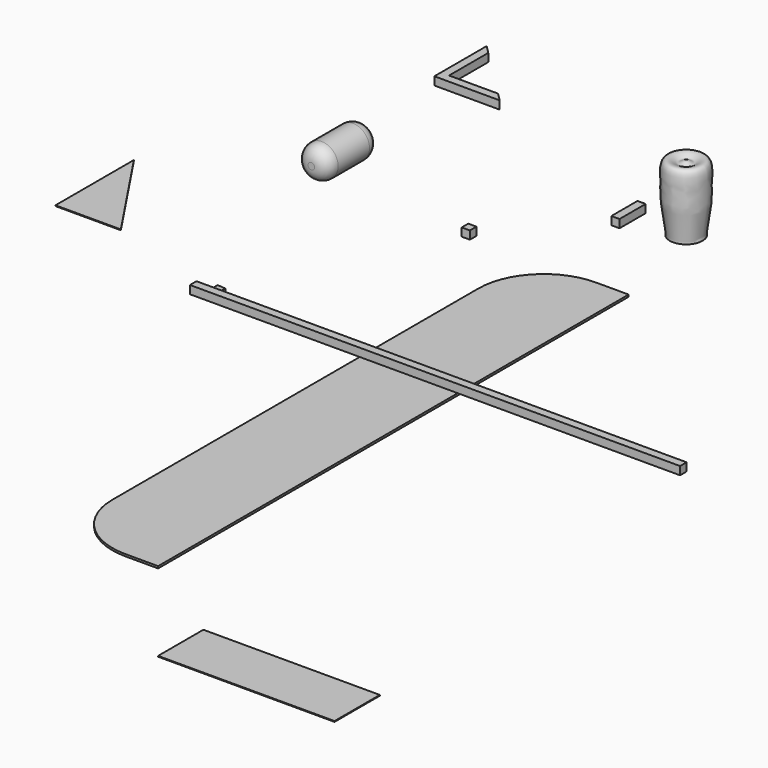
from build123d import *

# Parameters (mm, degrees)
F0_W      = 76.2
F0_H      = 1.5875
F1_DEPTH  = 457.2
F2_W      = 6.35
F2_H      = 6.35
F3_DEPTH  = 381
F4_W      = 44.45
F4_H      = 6.35
F5_DEPTH  = 6.35
F6_SIZE2  = 6.34999
F6_SIZE   = 6.34999
F7_SIZE2  = 6.34999
F7_SIZE   = 6.34999
F8_ANGLE  = 90
F9_W      = 6.35
F9_H      = 6.35
F10_DEPTH = 6.35
F11_R     = 50.8
F12_R     = 50.8
F13_W     = 137.16
F13_H     = 44.0000009
F14_DEPTH = 0.5999999938
F15_W     = 6.35
F15_H     = 6.35
F16_DEPTH = 25.4
F18_DEPTH = 0.5999999938
F20_DEPTH = 6.35
F21_R     = 12.7
F22_DEPTH = 50.8
F23_R     = 10.16
F24_R     = 10.16


# Not quite as in the source:
# - a fillet or chamfer is up to 0.001 mm smaller than in the source, because OpenCascade refuses the exact size


with BuildPart() as f1:
    # F0 (on Front) → F1 (new body)
    with BuildSketch(Plane.XZ):
        with Locations((27.2368646166, 23.0428799987)):
            Rectangle(F0_W, F0_H)
    extrude(amount=F1_DEPTH)

    # F11
    f11_edges = [f1.edges().sort_by_distance(p)[0] for p in [
        (-10.863135, -457.2, 23.04288),
    ]]
    fillet(f11_edges, radius=F11_R)

    # F12
    f12_edges = [f1.edges().sort_by_distance(p)[0] for p in [
        (-10.863135, 0, 23.04288),
    ]]
    fillet(f12_edges, radius=F12_R)


with BuildPart() as f3:
    # F2 (on Right) → F3 (new body)
    with BuildSketch(Plane.YZ):
        with Locations((-341.438638593, 146.0574641824)):
            Rectangle(F2_W, F2_H)
    extrude(amount=F3_DEPTH)


with BuildPart() as f5:
    # F4 (on Front) → F5 (new body)
    with BuildSketch(Plane.XZ):
        with Locations((-52.0163912032, 118.8257239481)):
            Rectangle(F4_W, F4_H)
        Polygon((-74.2413912032, 122.0007239481), (-80.5913912032, 122.0007239481), (-80.5913912032, 71.2007239481), (-74.2413912032, 71.2007239481), (-74.2413912032, 115.6507239481), align=None)
    extrude(amount=F5_DEPTH)

    # F6 (size 6.35 and 6.35 in the source; OpenCascade refuses exactly that, so slightly less here)
    f6_edges = [f5.edges().sort_by_distance(p)[0] for p in [
        (-29.791391, -3.175, 115.650724),
    ]]
    chamfer(f6_edges, length=F6_SIZE, length2=F6_SIZE2)

    # F7 (size 6.35 and 6.35 in the source; OpenCascade refuses exactly that, so slightly less here)
    f7_edges = [f5.edges().sort_by_distance(p)[0] for p in [
        (-74.241391, -3.175, 71.200724),
    ]]
    chamfer(f7_edges, length=F7_SIZE, length2=F7_SIZE2)


with BuildPart() as f5_1:
    # F8: moved
    add(f5.part.rotate(Axis((-55.1913912032, -6.35, 122.0007239481), (1, 0, 0)), F8_ANGLE))


with BuildPart() as f10:
    # F9 (on Front) → F10 (new body)
    with BuildSketch(Plane.XZ):
        with Locations((-56.1577156186, 28.6541397465)):
            Rectangle(F9_W, F9_H)
    extrude(amount=F10_DEPTH)


with BuildPart() as f14:
    # F13 (on Top) → F14 (new body)
    with BuildSketch(Plane.XY):
        with Locations((179.7031573951, -492.4447879232)):
            Rectangle(F13_W, F13_H)
    extrude(amount=F14_DEPTH)


with BuildPart() as f16:
    # F15 (on Front) → F16 (new body)
    with BuildSketch(Plane.XZ):
        with Locations((75.4093378782, 86.979034377)):
            Rectangle(F15_W, F15_H)
    extrude(amount=F16_DEPTH)


with BuildPart() as f18:
    # F17 (on Top) → F18 (new body)
    with BuildSketch(Plane.XY):
        Polygon((-307.5355387568, -14.609475274), (-307.5355387568, -90.809475274), (-256.7355387568, -90.809475274), align=None)
    extrude(amount=F18_DEPTH)


with BuildPart() as f20:
    # F19 (on Top) → F20 (new body)
    with BuildSketch(Plane.XY):
        Polygon((-158.2077033869, -119.8694149069), (-158.2077033869, -126.2194149069), (-151.8577033869, -126.2194149069), (-151.8577033869, -120.4249679203), align=None)
    extrude(amount=F20_DEPTH)


with BuildPart() as f22:
    # F21 (on Front) → F22 (new body)
    with BuildSketch(Plane.XZ):
        with Locations((-140.6690627337, 65.3587505221)):
            Circle(F21_R)
    extrude(amount=F22_DEPTH)

    # F23
    f23_edges = [f22.edges().sort_by_distance(p)[0] for p in [
        (-153.369063, -50.8, 65.358751),
    ]]
    fillet(f23_edges, radius=F23_R)

    # F24
    f24_edges = [f22.edges().sort_by_distance(p)[0] for p in [
        (-153.369063, 0, 65.358751),
    ]]
    fillet(f24_edges, radius=F24_R)


with BuildPart() as f26:
    # F25 (on Front) → F26 (revolve)
    with BuildSketch(Plane.XZ):
        with BuildLine():
            add(Edge.make_bspline(
                [(110.0819293248, 130.0819069862), (110.3717446977, 130.1103268683), (111.7587693127, 130.4941438289), (115.1430049235, 127.5772588495), (118.1984273121, 130.4327242695), (123.7508982405, 131.842131525), (126.5857018365, 126.1634027602), (125.5943246161, 115.0864014057), (126.5688541924, 103.9398980057), (122.0392190427, 82.2117755317), (122.7072343646, 79.8075409987), (122.7819293248, 79.2819069862)],
                knots=[0, 0, 0, 0, 0.0535265271, 0.1394449349, 0.2248612903, 0.3220822803, 0.4217359368, 0.5658998253, 0.7249103589, 0.9301240545, 1, 1, 1, 1], degree=3))
            Line((110.0819293248, 130.0819069862), (110.0819293248, 79.2819069862))
            Line((110.0819293248, 79.2819069862), (122.7819293248, 79.2819069862))
        make_face()
    revolve(axis=Axis((110.0819293248, 0, 104.6819069862), (0, 0, -1)))


solid = Compound([f1.part, f3.part, f5_1.part, f10.part, f14.part, f16.part, f18.part, f20.part, f22.part, f26.part])
